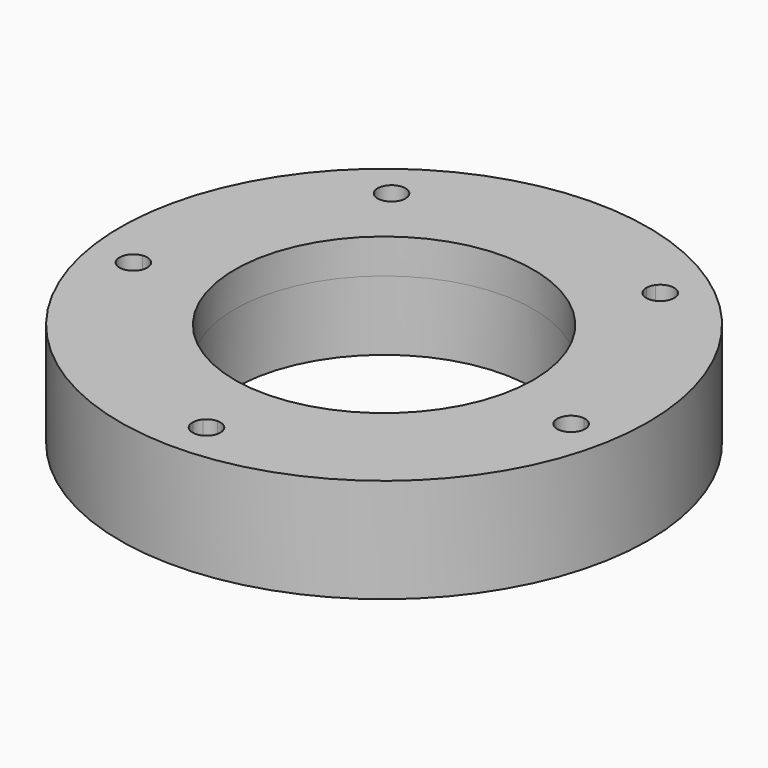
from build123d import *

# Parameters (mm, degrees)
F0_R     = 38
F0_R_2   = 21.5
F1_DEPTH = 10
F3_DEPTH = 10
F4_DEPTH = 5


with BuildPart() as f1:
    # F0 (on Top) → F1 (new body)
    with BuildSketch(Plane.XY):
        Circle(F0_R)
        Circle(F0_R_2, mode=Mode.SUBTRACT)
    extrude(amount=F1_DEPTH)

    # F2 (on face) → F3 (cut)
    with BuildSketch(Plane.XY.offset(10)):
        with BuildLine():
            ThreePointArc((17.3950694854, 25.5037771635), (18.7013512829, 23.576948176), (20.9465824354, 24.1917482683))
            ThreePointArc((20.9465824354, 24.1917482683), (19.3944253287, 25.4530207671), (17.7665087481, 26.6148674035))
            ThreePointArc((17.7665087481, 26.6148674035), (17.4976104485, 26.0871290467), (17.3950694854, 25.5037771635))
        make_face()
        with BuildLine():
            ThreePointArc((17.7665087481, 26.6148674035), (19.3944253287, 25.4530207671), (20.9465824354, 24.1917482683))
            ThreePointArc((20.9465824354, 24.1917482683), (21.2791420466, 24.7838101177), (21.3944253287, 25.4530207671))
            ThreePointArc((21.3944253287, 25.4530207671), (20.0044117379, 27.3577298212), (17.7665087481, 26.6148674035))
        make_face()
        with BuildLine():
            ThreePointArc((33.4880347509, -5.7011987796), (33.0028452429, -4.3953085953), (31.7826855775, -3.7230226271))
            ThreePointArc((31.7826855775, -3.7230226271), (31.6508184403, -4.7144132252), (31.4880347509, -5.7011987796))
            ThreePointArc((31.4880347509, -5.7011987796), (31.2944935166, -6.6824153971), (31.0703837886, -7.6571046244))
            ThreePointArc((31.0703837886, -7.6571046244), (32.7459493099, -7.2560785056), (33.4880347509, -5.7011987796))
        make_face()
        with BuildLine():
            ThreePointArc((31.4880347509, -5.7011987796), (31.6508184403, -4.7144132252), (31.7826855775, -3.7230226271))
            ThreePointArc((31.7826855775, -3.7230226271), (29.7436669076, -4.7228425934), (29.9536778777, -6.9840662652))
            Line((29.9536778777, -6.9840662652), (31.4880347509, -5.7011987796))
        make_face()
        with BuildLine():
            ThreePointArc((31.0703837886, -7.6571046244), (31.2944935166, -6.6824153971), (31.4880347509, -5.7011987796))
            Line((31.4880347509, -5.7011987796), (29.9536778777, -6.9840662652))
            ThreePointArc((29.9536778777, -6.9840662652), (30.4556448993, -7.414141042), (31.0703837886, -7.6571046244))
        make_face()
        with BuildLine():
            ThreePointArc((-17.3276317844, 25.5037771635), (-17.4221248046, 26.1112663816), (-17.6966749345, 26.6613521087))
            ThreePointArc((-17.6966749345, 26.6613521087), (-19.3276317844, 25.5037771635), (-20.8830900727, 24.2465780888))
            ThreePointArc((-20.8830900727, 24.2465780888), (-18.6608921713, 23.6181848724), (-17.3276317844, 25.5037771635))
        make_face()
        with BuildLine():
            ThreePointArc((-20.8830900727, 24.2465780888), (-19.3276317844, 25.5037771635), (-17.6966749345, 26.6613521087))
            ThreePointArc((-17.6966749345, 26.6613521087), (-20.5356087709, 27.0977632362), (-20.8830900727, 24.2465780888))
        make_face()
        with BuildLine():
            Line((0.0337188505, -31.999982235), (1.5680757237, -30.7171147494))
            ThreePointArc((1.5680757237, -30.7171147494), (0.8805556201, -30.1881137283), (0.0337188505, -29.999982235))
            Line((0.0337188505, -29.999982235), (0.0337188505, -31.999982235))
        make_face()
        with BuildLine():
            ThreePointArc((2.0326750825, -31.9353758708), (1.9024391118, -31.2873220179), (1.5680757237, -30.7171147494))
            Line((1.5680757237, -30.7171147494), (0.0337188505, -31.999982235))
            ThreePointArc((0.0337188505, -31.999982235), (1.033701827, -31.983299713), (2.0326750825, -31.9353758708))
        make_face()
        with BuildLine():
            ThreePointArc((2.0337188505, -31.999982235), (2.0334578915, -31.9676748374), (2.0326750825, -31.9353758708))
            ThreePointArc((2.0326750825, -31.9353758708), (1.033701827, -31.983299713), (0.0337188505, -31.999982235))
            ThreePointArc((0.0337188505, -31.999982235), (-0.9662970627, -31.9854071412), (-1.9653690958, -31.9395886686))
            ThreePointArc((-1.9653690958, -31.9395886686), (0.003518624, -33.9997542086), (2.0337188505, -31.999982235))
        make_face()
        with BuildLine():
            Line((0.0337188505, -31.999982235), (0.0337188505, -29.999982235))
            ThreePointArc((0.0337188505, -29.999982235), (-0.8150266404, -30.189007058), (-1.503338165, -30.7203511432))
            Line((-1.503338165, -30.7203511432), (0.0337188505, -31.999982235))
        make_face()
        with BuildLine():
            ThreePointArc((-1.9653690958, -31.9395886686), (-0.9662970627, -31.9854071412), (0.0337188505, -31.999982235))
            Line((0.0337188505, -31.999982235), (-1.503338165, -30.7203511432))
            ThreePointArc((-1.503338165, -30.7203511432), (-1.8364991405, -31.2912617919), (-1.9653690958, -31.9395886686))
        make_face()
        with BuildLine():
            ThreePointArc((-29.4759499676, -5.7675448535), (-30.1716566854, -4.2513591676), (-31.7747690017, -3.7899940488))
            ThreePointArc((-31.7747690017, -3.7899940488), (-31.640812874, -4.7811045451), (-31.4759499676, -5.7675448535))
            Line((-31.4759499676, -5.7675448535), (-29.9388929521, -7.0471759453))
            ThreePointArc((-29.9388929521, -7.0471759453), (-29.5952434473, -6.4479439896), (-29.4759499676, -5.7675448535))
        make_face()
        with BuildLine():
            ThreePointArc((-31.4759499676, -5.7675448535), (-31.640812874, -4.7811045451), (-31.7747690017, -3.7899940488))
            ThreePointArc((-31.7747690017, -3.7899940488), (-33.4431968406, -6.1280164068), (-31.054178004, -7.722566186))
            ThreePointArc((-31.054178004, -7.722566186), (-31.2803413207, -6.7483514181), (-31.4759499676, -5.7675448535))
        make_face()
        with BuildLine():
            Line((-29.9388929521, -7.0471759453), (-31.4759499676, -5.7675448535))
            ThreePointArc((-31.4759499676, -5.7675448535), (-31.2803413207, -6.7483514181), (-31.054178004, -7.722566186))
            ThreePointArc((-31.054178004, -7.722566186), (-30.4399525078, -7.4783076258), (-29.9388929521, -7.0471759453))
        make_face()
    extrude(amount=-F3_DEPTH, mode=Mode.SUBTRACT)

    # F4 (add): a face of the model
    f4_faces = [f1.faces().sort_by_distance(p)[0] for p in [
        (-36.9251976926, 0, 10),
    ]]
    extrude(f4_faces, amount=F4_DEPTH)


solid = f1.part
